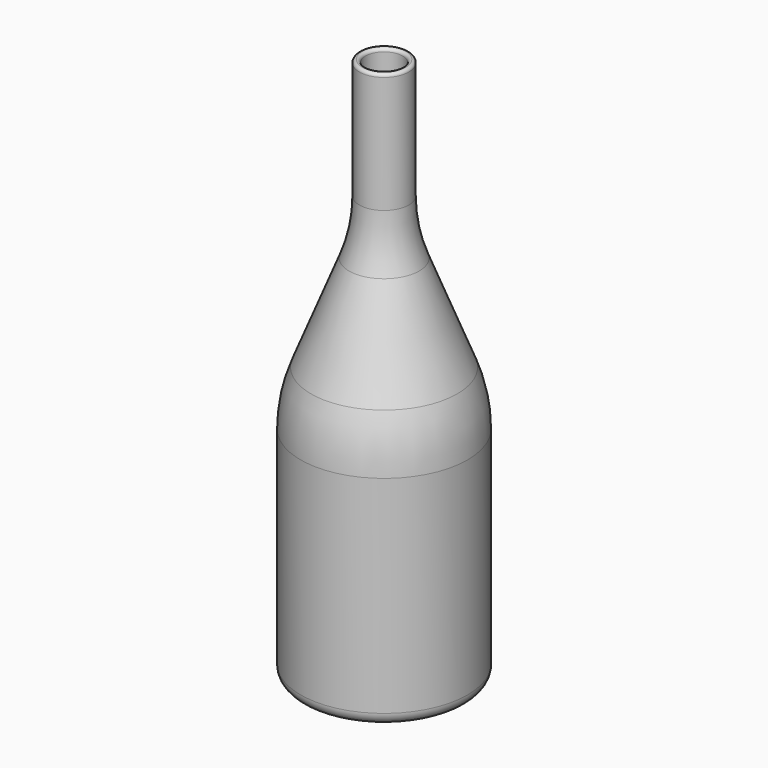
from build123d import *

# Parameters (mm, degrees)
F2_R = 1.58749


# Not quite as in the source:
# - a fillet or chamfer is up to 0.001 mm smaller than in the source, because OpenCascade refuses the exact size


with BuildPart() as f1:
    # F0 (on Front) → F1 (revolve)
    with BuildSketch(Plane.XZ):
        with BuildLine():
            Line((12.7, 152.5613266138), (9.525, 152.5613266138))
            Line((9.525, 152.5613266138), (9.525, 90.8940221579))
            ThreePointArc((9.525, 90.8940221579), (10.9303408592, 76.0238211347), (15.0966000875, 61.6801763592))
            Line((15.0966000875, 61.6801763592), (34.5616279195, 12.5053692045))
            ThreePointArc((34.5616279195, 12.5053692045), (38.3945864095, -0.6907839889), (39.6875, -14.3713689303))
            Line((39.6875, -14.3713689303), (39.6875, -117.3136733862))
            ThreePointArc((39.6875, -117.3136733862), (37.8276280605, -121.8038014467), (33.3375, -123.6636733862))
            Line((33.3375, -123.6636733862), (0, -123.6636733862))
            Line((0, -123.6636733862), (0, -126.8386733862))
            Line((0, -126.8386733862), (36.5125, -126.8386733862))
            ThreePointArc((36.5125, -126.8386733862), (41.0026280605, -124.9788014467), (42.8625, -120.4886733862))
            Line((42.8625, -120.4886733862), (42.8625, -14.3713689303))
            ThreePointArc((42.8625, -14.3713689303), (41.5133727751, -0.095975948), (37.513763916, 13.6739230365))
            Line((37.513763916, 13.6739230365), (18.048736084, 62.8487301912))
            ThreePointArc((18.048736084, 62.8487301912), (14.0491272249, 76.6186291756), (12.7, 90.8940221579))
            Line((12.7, 90.8940221579), (12.7, 152.5613266138))
        make_face()
    revolve(axis=Axis((0, 0, 12.8613266138), (0, 0, -1)))

    # F2 (radius 1.5875 in the source; OpenCascade refuses exactly that, so slightly less here)
    f2_edges = [f1.edges().sort_by_distance(p)[0] for p in [
        (-12.7, 0, 152.561327),
        (-9.525, 0, 152.561327),
    ]]
    fillet(f2_edges, radius=F2_R)


solid = f1.part
